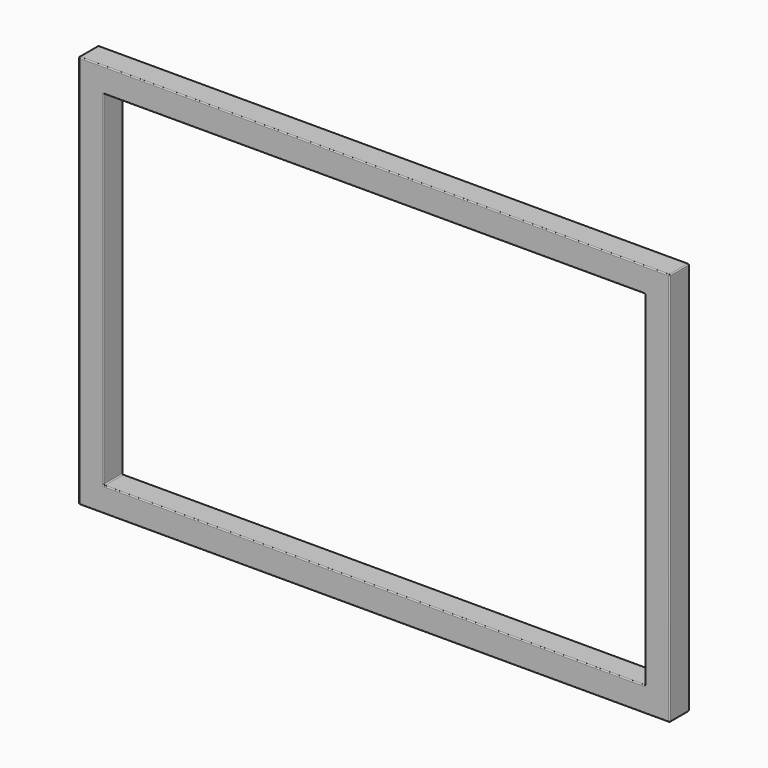
from build123d import *

# Parameters (mm, degrees)
F0_W     = 50
F0_H     = 700
F1_DEPTH = 50
F2_F1_R  = 2
F2_F2_R  = 2
F2_F3_R  = 2


with BuildPart() as f1:
    # F0 (on Front) → F1 (new body)
    with BuildSketch(Plane.XZ):
        Polygon((1200, 0), (0, 0), (0, -50), (50, -50), (1150, -50), (1200, -50), align=None)
        with Locations((25, -400)):
            Rectangle(F0_W, F0_H)
        Polygon((50, -750), (0, -750), (0, -800), (1200, -800), (1200, -750), (1150, -750), align=None)
        with Locations((1175, -400)):
            Rectangle(F0_W, F0_H)
    extrude(amount=F1_DEPTH)

    # F2: fillet of radius 2 on 22 edges, made by hand

    # F2_f1
    f2_f1_edges = [f1.edges().sort_by_distance(p)[0] for p in [
        (50, -25, -50),
        (1150, -25, -50),
        (1150, -25, -750),
        (50, -25, -750),
    ]]
    fillet(f2_f1_edges, radius=F2_F1_R)

    # F2_f2
    f2_f2_edges = [f1.edges().sort_by_distance(p)[0] for p in [
        (600, -50, 0),
        (1200, -25, 0),
        (1200, -50, -400),
        (1200, 0, -400),
        (600, 0, 0),
        (0, 0, -400),
        (600, 0, -800),
        (600, -50, -50),
        (600, -50, -750),
        (0, -25, -800),
        (1200, -25, -800),
        (600, -50, -800),
        (0, -25, 0),
        (0, -50, -400),
        (1149.4142135624, -50, -749.4142135624),
        (50.5857864376, -50, -749.4142135624),
        (50.5857864376, -50, -50.5857864376),
        (1149.4142135624, -50, -50.5857864376),
    ]]
    fillet(f2_f2_edges, radius=F2_F2_R)

    # F2_f3
    f2_f3_edges = [f1.edges().sort_by_distance(p)[0] for p in [
        (600, 0, -750),
        (50, 0, -400),
        (600, 0, -50),
        (1150, 0, -400),
        (1149.4142135624, 0, -50.5857864376),
        (1149.4142135624, 0, -749.4142135624),
        (50.5857864376, 0, -50.5857864376),
        (50.5857864376, 0, -749.4142135624),
    ]]
    fillet(f2_f3_edges, radius=F2_F3_R)


solid = f1.part
